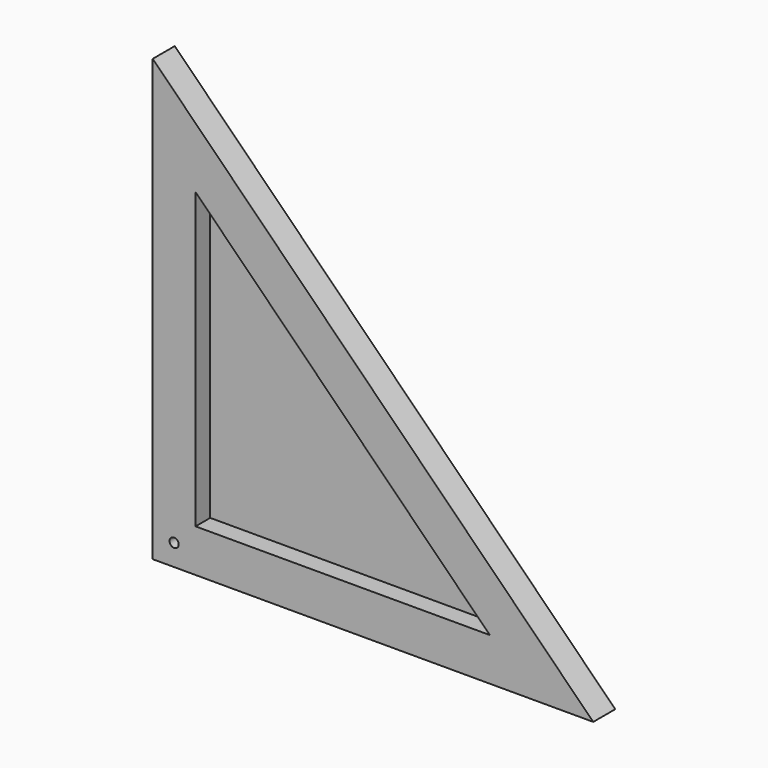
from build123d import *

# Parameters (mm, degrees)
F0_R     = 9.525
F1_DEPTH = 38.1
F2_DEPTH = 19.05


with BuildPart() as f1:
    # F0 (on Front) → F1 (new body)
    with BuildSketch(Plane.XZ):
        Polygon((914.4, 0), (0, 914.4), (0, 0), align=None)
        with Locations((44.45, 44.45)):
            Circle(F0_R, mode=Mode.SUBTRACT)
        Polygon((699.776414305, 88.9), (88.9, 88.9), (88.9, 699.776414305), align=None, mode=Mode.SUBTRACT)
    extrude(amount=F1_DEPTH)

    # F0 (on Front) → F2 (join)
    with BuildSketch(Plane.XZ):
        Polygon((914.4, 0), (0, 914.4), (0, 0), align=None)
        with Locations((44.45, 44.45)):
            Circle(F0_R, mode=Mode.SUBTRACT)
        Polygon((699.776414305, 88.9), (88.9, 88.9), (88.9, 699.776414305), align=None, mode=Mode.SUBTRACT)
        Polygon((88.9, 699.776414305), (88.9, 88.9), (699.776414305, 88.9), align=None)
    extrude(amount=-F2_DEPTH)


solid = f1.part
